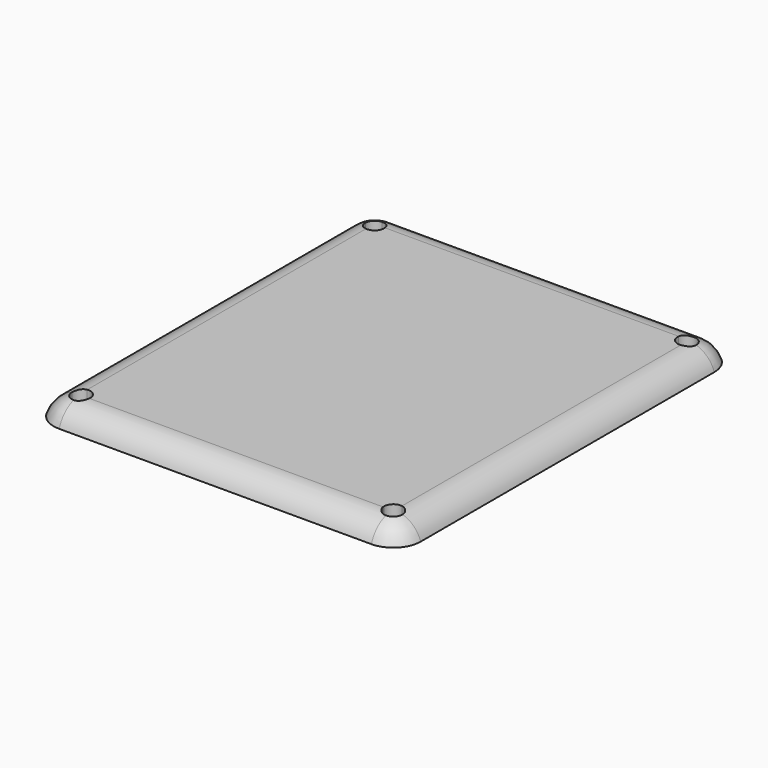
from build123d import *

# Parameters (mm, degrees)
F0_W         = 67
F0_H         = 77
F1_DEPTH     = 3.5
F2_R         = 5
F3_T1_DEPTH  = 57
F3_T3_DEPTH  = 67
F3_T6_ANGLE  = 90
F3_T8_ANGLE  = 90
F3_T10_ANGLE = 90
F3_T12_ANGLE = 90
F5_DEPTH     = 3.5


# Not quite as in the source:
# - a fillet or chamfer that OpenCascade refuses, or shapes differently, is made with other operations: its cross-section is extruded or revolved along the edge and cut away or added


with BuildPart() as f1:
    # F0 (on Top) → F1 (new body)
    with BuildSketch(Plane.XY):
        with Locations((33.5, -38.5)):
            Rectangle(F0_W, F0_H)
    extrude(amount=F1_DEPTH)

    # F2
    f2_edges = [f1.edges().sort_by_distance(p)[0] for p in [
        (67, -77, 1.75),
        (67, 0, 1.75),
        (0, 0, 1.75),
        (0, -77, 1.75),
    ]]
    fillet(f2_edges, radius=F2_R)

    # F3: fillet of radius 5 on 8 edges, made by hand

    # F3_s2 → F3_t1 (cut)
    with BuildSketch(Plane.YZ.offset(5)):
        with BuildLine():
            ThreePointArc((0, 0), (-1.8116561155, 2.5311288741), (-4.7696960071, 3.5))
            Line((-4.7696960071, 3.5), (0, 3.5))
            Line((0, 3.5), (0, 0))
        make_face()
        with BuildLine():
            ThreePointArc((-72.2303039929, 3.5), (-75.1883438845, 2.5311288741), (-77, 0))
            Line((-77, 0), (-77, 3.5))
            Line((-77, 3.5), (-72.2303039929, 3.5))
        make_face()
    extrude(amount=F3_T1_DEPTH, mode=Mode.SUBTRACT)

    # F3_s4 → F3_t3 (cut)
    with BuildSketch(Plane.XZ.offset(5)):
        with BuildLine():
            ThreePointArc((62.2303039929, 3.5), (65.1883438845, 2.5311288741), (67, 0))
            Line((67, 0), (67, 3.5))
            Line((67, 3.5), (62.2303039929, 3.5))
        make_face()
        with BuildLine():
            ThreePointArc((4.7696960071, 3.5), (1.8116561155, 2.5311288741), (0, 0))
            Line((0, 0), (0, 3.5))
            Line((0, 3.5), (4.7696960071, 3.5))
        make_face()
    extrude(amount=F3_T3_DEPTH, mode=Mode.SUBTRACT)

    # F3_s5 → F3_t6 (revolve, cut)
    with BuildSketch(Plane.YZ.offset(62)):
        with BuildLine():
            ThreePointArc((0, 0), (-1.8116561155, 2.5311288741), (-4.7696960071, 3.5))
            Line((-4.7696960071, 3.5), (0, 3.5))
            Line((0, 3.5), (0, 0))
        make_face()
    revolve(axis=Axis((62, -5, 3.5), (0, 0, -1)), revolution_arc=F3_T6_ANGLE, mode=Mode.SUBTRACT)

    # F3_s7 → F3_t8 (revolve, cut)
    with BuildSketch(Plane.YZ.offset(5)):
        with BuildLine():
            ThreePointArc((0, 0), (-1.8116561155, 2.5311288741), (-4.7696960071, 3.5))
            Line((-4.7696960071, 3.5), (0, 3.5))
            Line((0, 3.5), (0, 0))
        make_face()
    revolve(axis=Axis((5, -5, 3.5), (0, 0, 1)), revolution_arc=F3_T8_ANGLE, mode=Mode.SUBTRACT)

    # F3_s9 → F3_t10 (revolve, cut)
    with BuildSketch(Plane.YZ.offset(62)):
        with BuildLine():
            ThreePointArc((-72.2303039929, 3.5), (-75.1883438845, 2.5311288741), (-77, 0))
            Line((-77, 0), (-77, 3.5))
            Line((-77, 3.5), (-72.2303039929, 3.5))
        make_face()
    revolve(axis=Axis((62, -72, 3.5), (0, 0, 1)), revolution_arc=F3_T10_ANGLE, mode=Mode.SUBTRACT)

    # F3_s11 → F3_t12 (revolve, cut)
    with BuildSketch(Plane.XZ.offset(72)):
        with BuildLine():
            ThreePointArc((4.7696960071, 3.5), (1.8116561155, 2.5311288741), (0, 0))
            Line((0, 0), (0, 3.5))
            Line((0, 3.5), (4.7696960071, 3.5))
        make_face()
    revolve(axis=Axis((5, -72, 3.5), (0, 0, 1)), revolution_arc=F3_T12_ANGLE, mode=Mode.SUBTRACT)

    # F4 (on face) → F5 (cut)
    with BuildSketch(Plane.XY.offset(3.5)):
        with BuildLine():
            Line((62.2303039929, -72), (63.7, -72))
            ThreePointArc((63.7, -72), (63.5705952053, -71.349438165), (63.202081528, -70.797918472))
            Line((63.202081528, -70.797918472), (62.2303039929, -71.7696960071))
            Line((62.2303039929, -71.7696960071), (62.2303039929, -72))
        make_face()
        with BuildLine():
            ThreePointArc((63.202081528, -70.797918472), (62.7556933452, -70.4771974626), (62.2303039929, -70.3156722199))
            Line((62.2303039929, -70.3156722199), (62.2303039929, -71.7696960071))
            Line((62.2303039929, -71.7696960071), (63.202081528, -70.797918472))
        make_face()
        with BuildLine():
            ThreePointArc((62.2303039929, -70.3156722199), (60.8823052268, -70.7190790836), (60.3, -72))
            Line((60.3, -72), (62, -72))
            Line((62, -72), (62.2303039929, -71.7696960071))
            Line((62.2303039929, -71.7696960071), (62.2303039929, -70.3156722199))
        make_face()
        with BuildLine():
            Line((62, -72.2303039929), (60.3156722199, -72.2303039929))
            ThreePointArc((60.3156722199, -72.2303039929), (62.1154183127, -73.6960774195), (63.7, -72))
            Line((63.7, -72), (62.2303039929, -72))
            ThreePointArc((62.2303039929, -72), (62.1628495151, -72.1628495151), (62, -72.2303039929))
        make_face()
        with BuildLine():
            ThreePointArc((60.3, -72), (60.3039225805, -72.1154183127), (60.3156722199, -72.2303039929))
            Line((60.3156722199, -72.2303039929), (62, -72.2303039929))
            ThreePointArc((62, -72.2303039929), (62.1628495151, -72.1628495151), (62.2303039929, -72))
            Line((62.2303039929, -72), (62, -72))
            Line((62, -72), (60.3, -72))
        make_face()
        Polygon((62.2303039929, -71.7696960071), (62, -72), (62.2303039929, -72), align=None)
        with BuildLine():
            Line((4.7696960071, -72), (3.3, -72))
            ThreePointArc((3.3, -72), (4.8845816873, -73.6960774195), (6.6843277801, -72.2303039929))
            Line((6.6843277801, -72.2303039929), (5, -72.2303039929))
            ThreePointArc((5, -72.2303039929), (4.8371504849, -72.1628495151), (4.7696960071, -72))
        make_face()
        with BuildLine():
            ThreePointArc((4.7696960071, -70.3156722199), (3.7190790836, -70.8823052268), (3.3, -72))
            Line((3.3, -72), (4.7696960071, -72))
            Line((4.7696960071, -72), (4.7696960071, -70.3156722199))
        make_face()
        with BuildLine():
            Line((4.7696960071, -70.3156722199), (4.7696960071, -72))
            Line((4.7696960071, -72), (6.7, -72))
            ThreePointArc((6.7, -72), (6.1176947732, -70.7190790836), (4.7696960071, -70.3156722199))
        make_face()
        with BuildLine():
            Line((6.7, -72), (4.7696960071, -72))
            ThreePointArc((4.7696960071, -72), (4.8371504849, -72.1628495151), (5, -72.2303039929))
            Line((5, -72.2303039929), (6.6843277801, -72.2303039929))
            ThreePointArc((6.6843277801, -72.2303039929), (6.6960774195, -72.1154183127), (6.7, -72))
        make_face()
        with BuildLine():
            Line((5, -4.7696960071), (5, -3.3))
            ThreePointArc((5, -3.3), (3.797918472, -3.797918472), (3.3, -5))
            Line((3.3, -5), (4.7696960071, -5))
            ThreePointArc((4.7696960071, -5), (4.8371504849, -4.8371504849), (5, -4.7696960071))
        make_face()
        with BuildLine():
            ThreePointArc((6.6843277801, -4.7696960071), (6.1176947732, -3.7190790836), (5, -3.3))
            Line((5, -3.3), (5, -4.7696960071))
            Line((5, -4.7696960071), (6.6843277801, -4.7696960071))
        make_face()
        with BuildLine():
            Line((6.6843277801, -4.7696960071), (5, -4.7696960071))
            Line((5, -4.7696960071), (5, -5))
            Line((5, -5), (4.7696960071, -5))
            Line((4.7696960071, -5), (4.7696960071, -6.6843277801))
            ThreePointArc((4.7696960071, -6.6843277801), (6.1176947732, -6.2809209164), (6.7, -5))
            ThreePointArc((6.7, -5), (6.6960774195, -4.8845816873), (6.6843277801, -4.7696960071))
        make_face()
        with BuildLine():
            Line((4.7696960071, -5), (3.3, -5))
            ThreePointArc((3.3, -5), (3.7190790836, -6.1176947732), (4.7696960071, -6.6843277801))
            Line((4.7696960071, -6.6843277801), (4.7696960071, -5))
        make_face()
        with BuildLine():
            Line((5, -5), (5, -4.7696960071))
            ThreePointArc((5, -4.7696960071), (4.8371504849, -4.8371504849), (4.7696960071, -5))
            Line((4.7696960071, -5), (5, -5))
        make_face()
        with BuildLine():
            Line((62, -4.7696960071), (60.3156722199, -4.7696960071))
            ThreePointArc((60.3156722199, -4.7696960071), (60.797918472, -6.202081528), (62.2303039929, -6.6843277801))
            Line((62.2303039929, -6.6843277801), (62.2303039929, -5))
            ThreePointArc((62.2303039929, -5), (62.1628495151, -4.8371504849), (62, -4.7696960071))
        make_face()
        with BuildLine():
            ThreePointArc((63.7, -5), (62.1154183127, -3.3039225805), (60.3156722199, -4.7696960071))
            Line((60.3156722199, -4.7696960071), (62, -4.7696960071))
            ThreePointArc((62, -4.7696960071), (62.1628495151, -4.8371504849), (62.2303039929, -5))
            Line((62.2303039929, -5), (62.2303039929, -6.6843277801))
            ThreePointArc((62.2303039929, -6.6843277801), (63.2809209164, -6.1176947732), (63.7, -5))
        make_face()
    extrude(amount=-F5_DEPTH, mode=Mode.SUBTRACT)


solid = f1.part
